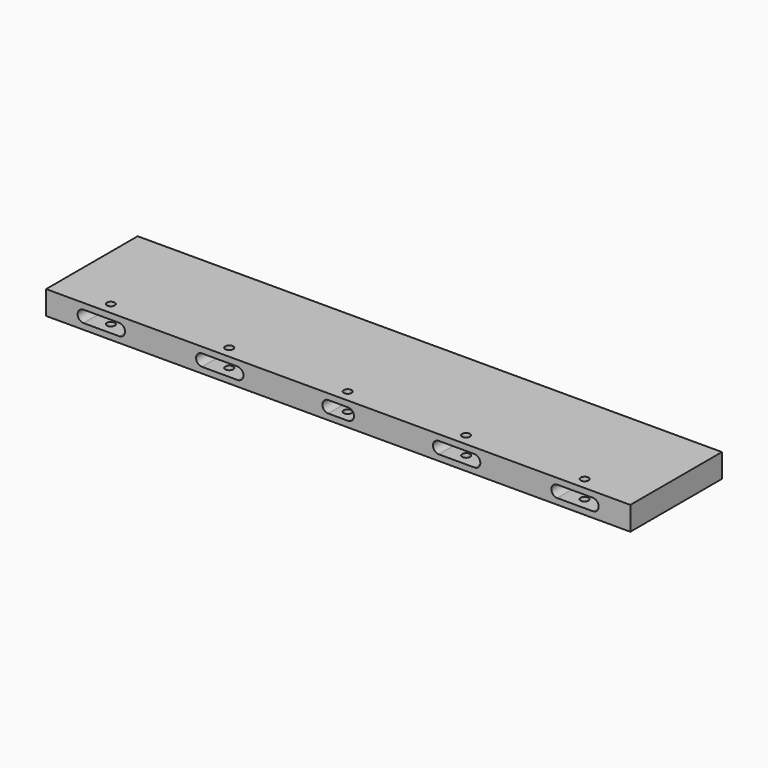
from build123d import *

# Parameters (mm, degrees)
F0_W     = 184.15
F0_H     = 38.1
F1_DEPTH = 939.8
F3_DEPTH = 38.1
F4_R     = 6.35
F5_DEPTH = 38.101


# Not quite as in the source:
# - a feature names something its author has since deleted; it is built from what else it names


with BuildPart() as f1:
    # F0 (on Right) → F1 (new body)
    with BuildSketch(Plane.YZ):
        with Locations((1.8085447712, 0)):
            Rectangle(F0_W, F0_H)
    extrude(amount=F1_DEPTH)

    # F2 (on face) → F3 (cut)
    with BuildSketch(Plane.XZ.offset(90.2664552288)):
        with BuildLine():
            Line((117.475, 9.525), (60.325, 9.525))
            ThreePointArc((60.325, 9.525), (50.8, 0), (60.325, -9.525))
            Line((60.325, -9.525), (117.475, -9.525))
            ThreePointArc((117.475, -9.525), (127, 0), (117.475, 9.525))
        make_face()
        with BuildLine():
            Line((307.975, 9.525), (250.825, 9.525))
            ThreePointArc((250.825, 9.525), (241.3, 0), (250.825, -9.525))
            Line((250.825, -9.525), (307.975, -9.525))
            ThreePointArc((307.975, -9.525), (317.5, 0), (307.975, 9.525))
        make_face()
        with BuildLine():
            Line((688.975, 9.525), (631.825, 9.525))
            ThreePointArc((631.825, 9.525), (622.3, 0), (631.825, -9.525))
            Line((631.825, -9.525), (688.975, -9.525))
            ThreePointArc((688.975, -9.525), (698.5, 0), (688.975, 9.525))
        make_face()
        with BuildLine():
            Line((879.475, 9.525), (822.325, 9.525))
            ThreePointArc((822.325, 9.525), (812.8, 0), (822.325, -9.525))
            Line((822.325, -9.525), (879.475, -9.525))
            ThreePointArc((879.475, -9.525), (889, 0), (879.475, 9.525))
        make_face()
        with BuildLine():
            Line((485.775, 9.525), (454.025, 9.525))
            ThreePointArc((454.025, 9.525), (444.5, 0), (454.025, -9.525))
            Line((454.025, -9.525), (485.775, -9.525))
            ThreePointArc((485.775, -9.525), (495.3, 0), (485.775, 9.525))
        make_face()
    extrude(amount=-F3_DEPTH, mode=Mode.SUBTRACT)

    # F4 (on face) → F5 (cut, through all)
    with BuildSketch(Plane.XY.offset(19.05)):
        with Locations((88.9, -71.2164552288)):
            Circle(F4_R)
        with Locations((279.4, -71.2164552288)):
            Circle(F4_R)
        with Locations((469.9, -71.2164552288)):
            Circle(F4_R)
        with Locations((660.4, -71.2164552288)):
            Circle(F4_R)
        with Locations((850.9, -71.2164552288)):
            Circle(F4_R)
    extrude(amount=-F5_DEPTH, mode=Mode.SUBTRACT)


solid = f1.part
